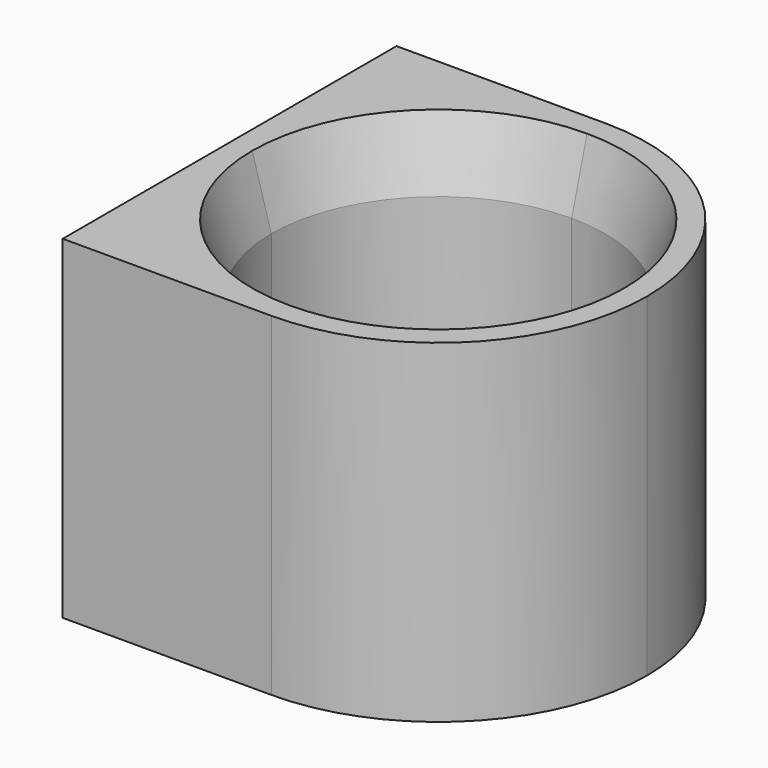
from build123d import *

# Parameters (mm, degrees)
F1_DEPTH = 25.4
F2_R     = 12.7
F3_DEPTH = 3.175
F5_DEPTH = 12.7
F6_SIZE2 = 1.4566665597
F6_SIZE  = 5.08


with BuildPart() as f1:
    # F0 (on Top) → F1 (new body)
    with BuildSketch(Plane.XY):
        with BuildLine():
            ThreePointArc((-15.875, 0), (-11.2253201513, 11.2253201513), (0, 15.875))
            Line((0, 15.875), (-15.875, 15.875))
            Line((-15.875, 15.875), (-15.875, 0))
        make_face()
        with BuildLine():
            Line((-15.875, -15.875), (0, -15.875))
            ThreePointArc((0, -15.875), (-11.2253201513, -11.2253201513), (-15.875, 0))
            Line((-15.875, 0), (-15.875, -15.875))
        make_face()
        with BuildLine():
            Line((0, -15.875), (0, -12.7))
            ThreePointArc((0, -12.7), (-8.9802561211, -8.9802561211), (-12.7, 0))
            Line((-12.7, 0), (-15.875, 0))
            ThreePointArc((-15.875, 0), (-11.2253201513, -11.2253201513), (0, -15.875))
        make_face()
        with BuildLine():
            ThreePointArc((-12.7, 0), (-8.9802561211, 8.9802561211), (0, 12.7))
            Line((0, 12.7), (0, 15.875))
            ThreePointArc((0, 15.875), (-11.2253201513, 11.2253201513), (-15.875, 0))
            Line((-15.875, 0), (-12.7, 0))
        make_face()
        with BuildLine():
            ThreePointArc((0, 12.7), (8.9802561211, 8.9802561211), (12.7, 0))
            ThreePointArc((12.7, 0), (8.9802561211, -8.9802561211), (0, -12.7))
            Line((0, -12.7), (0, -15.875))
            ThreePointArc((0, -15.875), (11.2253201513, -11.2253201513), (15.875, 0))
            ThreePointArc((15.875, 0), (11.2253201513, 11.2253201513), (0, 15.875))
            Line((0, 15.875), (0, 12.7))
        make_face()
    extrude(amount=F1_DEPTH)

    # F2 (on face) → F3 (join)
    with BuildSketch(Plane(origin=(0, 0, 0), x_dir=(1, 0, 0), z_dir=(0, 0, -1))):
        with BuildLine():
            Line((-15.875, 15.875), (-15.875, -15.875))
            Line((-15.875, -15.875), (0, -15.875))
            ThreePointArc((0, -15.875), (15.875, 0), (0, 15.875))
            Line((0, 15.875), (-15.875, 15.875))
        make_face()
        Circle(F2_R, mode=Mode.SUBTRACT)
        Circle(F2_R)
    extrude(amount=-F3_DEPTH)

    # F4 (on face) → F5 (cut)
    with BuildSketch(Plane(origin=(-15.875, 0, 0), x_dir=(0, -1, 0), z_dir=(-1, 0, 0))):
        Polygon((0, 6.35), (0, 9.525), (-7.9375, 9.525), (-11.90625, 9.525), (-11.90625, 6.35), (-7.9375, 6.35), align=None)
        Polygon((7.9375, 9.525), (0, 9.525), (0, 6.35), (7.9375, 6.35), (11.90625, 6.35), (11.90625, 9.525), align=None)
    extrude(amount=-F5_DEPTH, mode=Mode.SUBTRACT)

    # F6
    f6_edges = [f1.edges().sort_by_distance(p)[0] for p in [
        (0, -12.7, 25.4),
    ]]
    f6_side = f1.faces().sort_by_distance((0, -12.7, 14.2875))[0]
    chamfer(f6_edges, length=F6_SIZE, length2=F6_SIZE2, reference=f6_side)


solid = f1.part
